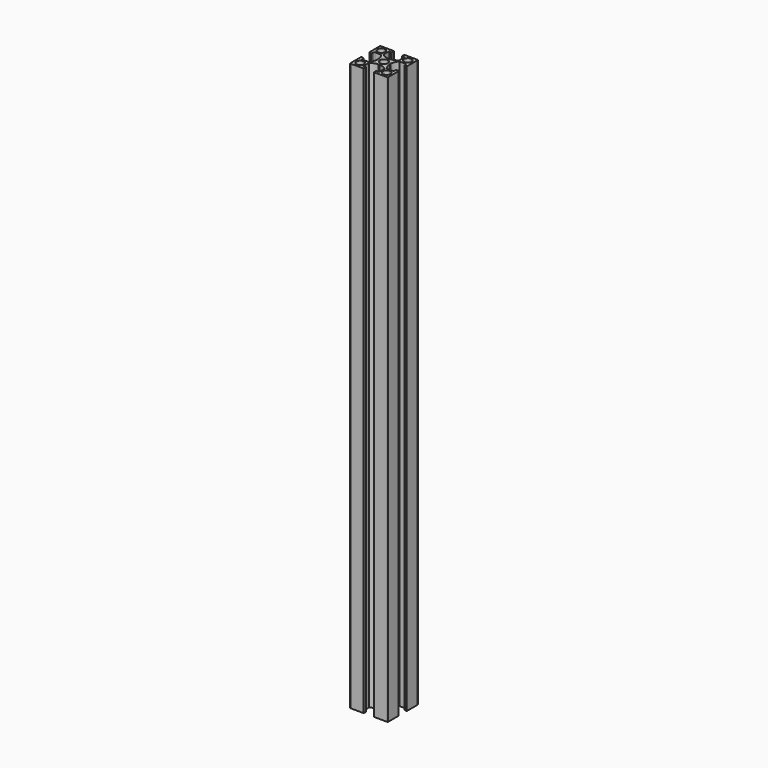
from build123d import *

# Parameters (mm, degrees)
F1_DEPTH = 300


# Not quite as in the source:
# - ends of sketch curves that miss each other by under 0.0002 mm in the source are joined


with BuildPart() as f1:
    # F0 (on Top) → F1 (new body)
    with BuildSketch(Plane.XY):
        with BuildLine():
            ThreePointArc((0, 2.15), (1.5202795796, 1.5202795796), (2.15, 0))
            Line((2.15, 0), (3, 0))
            Line((3, 0), (3.307278, 0.307278))
            ThreePointArc((3.307278, 0.307278), (3.7143803747, 2.2820219924), (4.7078187099, 4.0365664363))
            ThreePointArc((4.7078187099, 4.0365664363), (4.812308461, 4.1201573706), (4.94275, 4.15))
            Line((4.94275, 4.15), (8.2, 4.15))
            ThreePointArc((8.2, 4.15), (8.4121320344, 4.0621320344), (8.5, 3.85))
            Line((8.5, 3.85), (8.5, 2.95))
            ThreePointArc((8.5, 2.95), (8.5878679656, 2.7378679656), (8.8, 2.65))
            Line((8.8, 2.65), (9.7, 2.65))
            ThreePointArc((9.7, 2.65), (9.9121320344, 2.7378679656), (10, 2.95))
            Line((10, 2.95), (10, 9.7))
            ThreePointArc((10, 9.7), (9.9121320344, 9.9121320344), (9.7, 10))
            Line((9.7, 10), (2.95, 10))
            ThreePointArc((2.95, 10), (2.7378679656, 9.9121320344), (2.65, 9.7))
            Line((2.65, 9.7), (2.65, 8.8))
            ThreePointArc((2.65, 8.8), (2.7378679656, 8.5878679656), (2.95, 8.5))
            Line((2.95, 8.5), (3.85, 8.5))
            ThreePointArc((3.85, 8.5), (4.0621320344, 8.4121320344), (4.15, 8.2))
            Line((4.15, 8.2), (4.15, 4.94275))
            ThreePointArc((4.15, 4.94275), (4.1201572004, 4.8123081084), (4.036566086, 4.7078178916))
            ThreePointArc((4.036566086, 4.7078178916), (2.2820216259, 3.7143802371), (0.3072779813, 3.3072783955))
            Line((0.3072779813, 3.3072783955), (0, 3))
            Line((0, 3), (0, 2.15))
        make_face()
        with BuildLine():
            ThreePointArc((7, 9), (8.4142135624, 8.4142135624), (9, 7))
            ThreePointArc((9, 7), (8.4142135624, 5.5857864376), (7, 5))
            ThreePointArc((7, 5), (5.5857864376, 5.5857864376), (5, 7))
            ThreePointArc((5, 7), (5.5857864376, 8.4142135624), (7, 9))
        make_face(mode=Mode.SUBTRACT)
        with BuildLine():
            Line((3, 0), (2.15, 0))
            ThreePointArc((2.15, 0), (1.5202795796, -1.5202795796), (0, -2.15))
            Line((0, -2.15), (0, -3))
            Line((0, -3), (0.307278, -3.307277))
            ThreePointArc((0.307278, -3.307277), (2.2820216259, -3.7143792371), (4.036565823, -4.7078172229))
            ThreePointArc((4.036565823, -4.7078172229), (4.1201572004, -4.8123071084), (4.15, -4.942749))
            Line((4.15, -4.942749), (4.15, -8.2))
            ThreePointArc((4.15, -8.2), (4.0621320344, -8.4121320344), (3.85, -8.5))
            Line((3.85, -8.5), (2.95, -8.5))
            ThreePointArc((2.95, -8.5), (2.7378679656, -8.5878679656), (2.65, -8.8))
            Line((2.65, -8.8), (2.65, -9.7))
            ThreePointArc((2.65, -9.7), (2.7378679656, -9.9121320344), (2.95, -10))
            Line((2.95, -10), (9.7, -10))
            ThreePointArc((9.7, -10), (9.9121320344, -9.9121320344), (10, -9.7))
            Line((10, -9.7), (10, -2.95))
            ThreePointArc((10, -2.95), (9.9121320344, -2.7378679656), (9.7, -2.65))
            Line((9.7, -2.65), (8.8, -2.65))
            ThreePointArc((8.8, -2.65), (8.5878679656, -2.7378679656), (8.5, -2.95))
            Line((8.5, -2.95), (8.5, -3.85))
            ThreePointArc((8.5, -3.85), (8.4121320344, -4.0621320344), (8.2, -4.15))
            Line((8.2, -4.15), (4.94275, -4.15))
            ThreePointArc((4.94275, -4.15), (4.8123081084, -4.1201572004), (4.7078178916, -4.036566086))
            ThreePointArc((4.7078178916, -4.036566086), (3.7143800615, -2.2820211583), (3.3072783483, -0.3072769835))
            Line((3.3072783483, -0.3072769835), (3, 0))
        make_face()
        with BuildLine():
            ThreePointArc((7, -5), (8.4142135624, -5.5857864376), (9, -7))
            ThreePointArc((9, -7), (8.4142135624, -8.4142135624), (7, -9))
            ThreePointArc((7, -9), (5.5857864376, -8.4142135624), (5, -7))
            ThreePointArc((5, -7), (5.5857864376, -5.5857864376), (7, -5))
        make_face(mode=Mode.SUBTRACT)
        with BuildLine():
            ThreePointArc((-2.15, 0), (-1.5202795796, 1.5202795796), (0, 2.15))
            Line((0, 2.15), (0, 3))
            Line((0, 3), (-0.307277, 3.307278))
            ThreePointArc((-0.307277, 3.307278), (-2.2820211583, 3.7143800615), (-4.036565823, 4.7078182229))
            ThreePointArc((-4.036565823, 4.7078182229), (-4.1201572004, 4.8123081084), (-4.15, 4.94275))
            Line((-4.15, 4.94275), (-4.15, 8.2))
            ThreePointArc((-4.15, 8.2), (-4.0621320344, 8.4121320344), (-3.85, 8.5))
            Line((-3.85, 8.5), (-2.95, 8.5))
            ThreePointArc((-2.95, 8.5), (-2.7378679656, 8.5878679656), (-2.65, 8.8))
            Line((-2.65, 8.8), (-2.65, 9.7))
            ThreePointArc((-2.65, 9.7), (-2.7378679656, 9.9121320344), (-2.95, 10))
            Line((-2.95, 10), (-9.7, 10))
            ThreePointArc((-9.7, 10), (-9.9121320344, 9.9121320344), (-10, 9.7))
            Line((-10, 9.7), (-10, 2.95))
            ThreePointArc((-10, 2.95), (-9.9121320344, 2.7378679656), (-9.7, 2.65))
            Line((-9.7, 2.65), (-8.8, 2.65))
            ThreePointArc((-8.8, 2.65), (-8.5878679656, 2.7378679656), (-8.5, 2.95))
            Line((-8.5, 2.95), (-8.5, 3.85))
            ThreePointArc((-8.5, 3.85), (-8.4121320344, 4.0621320344), (-8.2, 4.15))
            Line((-8.2, 4.15), (-4.942749, 4.15))
            ThreePointArc((-4.942749, 4.15), (-4.812307461, 4.1201573706), (-4.7078173786, 4.0365666993))
            ThreePointArc((-4.7078173786, 4.0365666993), (-3.7143793747, 2.2820219924), (-3.3072773955, 0.3072779813))
            Line((-3.3072773955, 0.3072779813), (-3, 0))
            Line((-3, 0), (-2.15, 0))
        make_face()
        with BuildLine():
            ThreePointArc((-7, 5), (-8.4142135624, 5.5857864376), (-9, 7))
            ThreePointArc((-9, 7), (-8.4142135624, 8.4142135624), (-7, 9))
            ThreePointArc((-7, 9), (-5.5857864376, 8.4142135624), (-5, 7))
            ThreePointArc((-5, 7), (-5.5857864376, 5.5857864376), (-7, 5))
        make_face(mode=Mode.SUBTRACT)
        with BuildLine():
            Line((0, -3), (0, -2.15))
            ThreePointArc((0, -2.15), (-1.5202795796, -1.5202795796), (-2.15, 0))
            Line((-2.15, 0), (-3, 0))
            Line((-3, 0), (-3.307277, -0.307277))
            ThreePointArc((-3.307277, -0.307277), (-3.7143790615, -2.2820211583), (-4.7078172229, -4.036565823))
            ThreePointArc((-4.7078172229, -4.036565823), (-4.8123071084, -4.1201572004), (-4.942749, -4.15))
            Line((-4.942749, -4.15), (-8.2, -4.15))
            ThreePointArc((-8.2, -4.15), (-8.4121320344, -4.0621320344), (-8.5, -3.85))
            Line((-8.5, -3.85), (-8.5, -2.95))
            ThreePointArc((-8.5, -2.95), (-8.5878679656, -2.7378679656), (-8.8, -2.65))
            Line((-8.8, -2.65), (-9.7, -2.65))
            ThreePointArc((-9.7, -2.65), (-9.9121320344, -2.7378679656), (-10, -2.95))
            Line((-10, -2.95), (-10, -9.7))
            ThreePointArc((-10, -9.7), (-9.9121320344, -9.9121320344), (-9.7, -10))
            Line((-9.7, -10), (-2.95, -10))
            ThreePointArc((-2.95, -10), (-2.7378679656, -9.9121320344), (-2.65, -9.7))
            Line((-2.65, -9.7), (-2.65, -8.8))
            ThreePointArc((-2.65, -8.8), (-2.7378679656, -8.5878679656), (-2.95, -8.5))
            Line((-2.95, -8.5), (-3.85, -8.5))
            ThreePointArc((-3.85, -8.5), (-4.0621320344, -8.4121320344), (-4.15, -8.2))
            Line((-4.15, -8.2), (-4.15, -4.942749))
            ThreePointArc((-4.15, -4.942749), (-4.1201572004, -4.8123071084), (-4.036566086, -4.7078168916))
            ThreePointArc((-4.036566086, -4.7078168916), (-2.2820211583, -3.7143790615), (-0.3072769835, -3.3072773483))
            Line((-0.3072769835, -3.3072773483), (0, -3))
        make_face()
        with BuildLine():
            ThreePointArc((-7, -9), (-8.4142135624, -8.4142135624), (-9, -7))
            ThreePointArc((-9, -7), (-8.4142135624, -5.5857864376), (-7, -5))
            ThreePointArc((-7, -5), (-5.5857864376, -5.5857864376), (-5, -7))
            ThreePointArc((-5, -7), (-5.5857864376, -8.4142135624), (-7, -9))
        make_face(mode=Mode.SUBTRACT)
    extrude(amount=F1_DEPTH)


solid = f1.part
